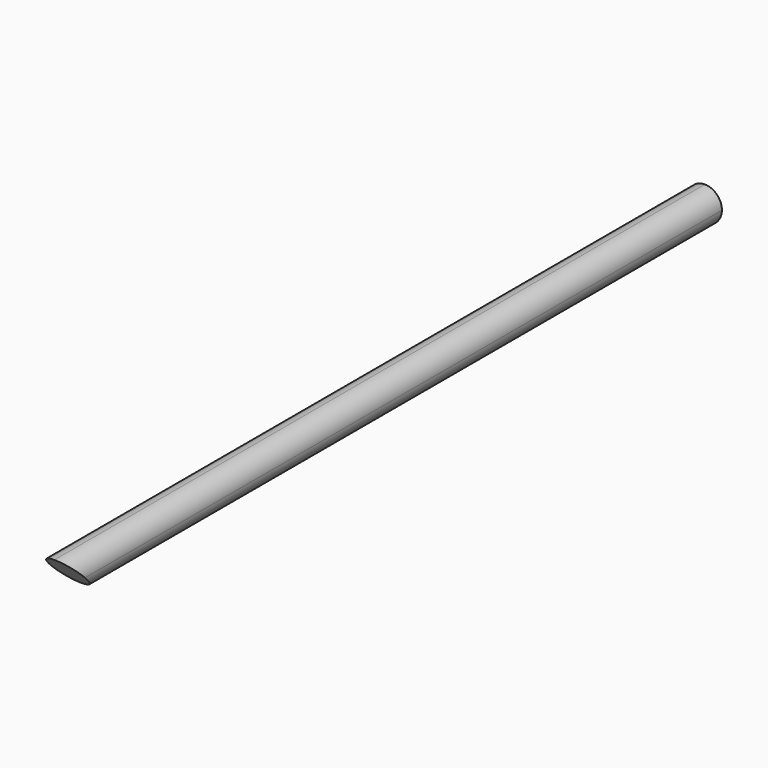
from build123d import *

# Parameters (mm, degrees)
F0_W     = 42
F0_H     = 42
F1_DEPTH = 1000
F3_DEPTH = 100
F4_R     = 20.99999


# Not quite as in the source:
# - a fillet or chamfer is up to 0.001 mm smaller than in the source, because OpenCascade refuses the exact size


with BuildPart() as f1:
    # F0 (on Front) → F1 (new body)
    with BuildSketch(Plane.XZ):
        Rectangle(F0_W, F0_H)
    extrude(amount=F1_DEPTH)

    # F2 (on face) → F3 (cut)
    with BuildSketch(Plane.YZ.offset(21)):
        Polygon((-958, -21), (-1000, 21), (-1000, -21), align=None)
    extrude(amount=-F3_DEPTH, mode=Mode.SUBTRACT)

    # F4 (radius 21 in the source; OpenCascade refuses exactly that, so slightly less here)
    f4_edges = [f1.edges().sort_by_distance(p)[0] for p in [
        (21, -500, 21),
        (21, -479, -21),
        (-21, -479, -21),
        (-21, -500, 21),
    ]]
    fillet(f4_edges, radius=F4_R)


solid = f1.part
